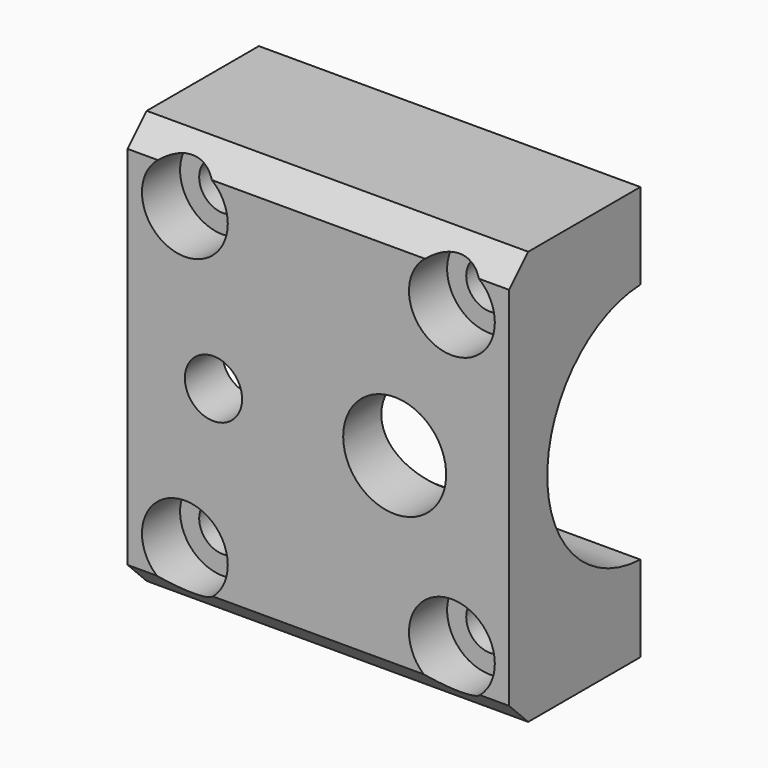
from build123d import *

# Parameters (mm, degrees)
F1_DEPTH       = 40
F3_D           = 5
F3_CBORE_D     = 9
F3_CBORE_DEPTH = 5
F4_T1_DEPTH    = 52.8584149398
F5_R           = 3
F6_DEPTH       = 17.201
F8_D           = 10.8
F8_DEPTH       = 11.35
F8_TIP         = 3.2446473427


# Not quite as in the source:
# - a fillet or chamfer that OpenCascade refuses, or shapes differently, is made with other operations: its cross-section is extruded or revolved along the edge and cut away or added


with BuildPart() as f1:
    # F0 (on Right) → F1 (new body)
    with BuildSketch(Plane.YZ):
        with BuildLine():
            ThreePointArc((-0.5, -12.6901536634), (-12.7, 0), (-0.5, 12.6901536634))
            Line((-0.5, 12.6901536634), (-0.5, 21.7))
            Line((-0.5, 21.7), (-17.7, 21.7))
            Line((-17.7, 21.7), (-17.7, -21.7))
            Line((-17.7, -21.7), (-0.5, -21.7))
            Line((-0.5, -21.7), (-0.5, -12.6901536634))
        make_face()
    extrude(amount=F1_DEPTH)

    # F3 (through all)
    with Locations(Plane.XZ.offset(17.7)):
        with Locations((6, 15.7), (34, 15.7), (34, -15.8), (6, -15.8)):
            CounterBoreHole(F3_D / 2, F3_CBORE_D / 2, F3_CBORE_DEPTH)

    # F4: chamfer of 2.5 on 2 edges, made by hand

    # F4_s2 → F4_t1 (cut)
    with BuildSketch(Plane.YZ.offset(-6.4292074699)):
        Polygon((-15.2, 21.7), (-17.7, 19.2), (-17.7, 21.7), align=None)
        Polygon((-15.2, -21.7), (-17.7, -19.2), (-17.7, -21.7), align=None)
    extrude(amount=F4_T1_DEPTH, mode=Mode.SUBTRACT)

    # F5 (on face) → F6 (cut, through all)
    with BuildSketch(Plane.XZ.offset(17.7)):
        with Locations((9, 0)):
            Circle(F5_R)
    extrude(amount=-F6_DEPTH, mode=Mode.SUBTRACT)

    # F8
    with Locations(Plane.XZ.offset(17.7)):
        with Locations((28, 0)):
            Hole(F8_D / 2, depth=F8_DEPTH)
            with Locations((0, 0, -(F8_DEPTH + F8_TIP / 2))):  # 118° drill point
                Cone(0, F8_D / 2, F8_TIP, mode=Mode.SUBTRACT)


solid = f1.part
